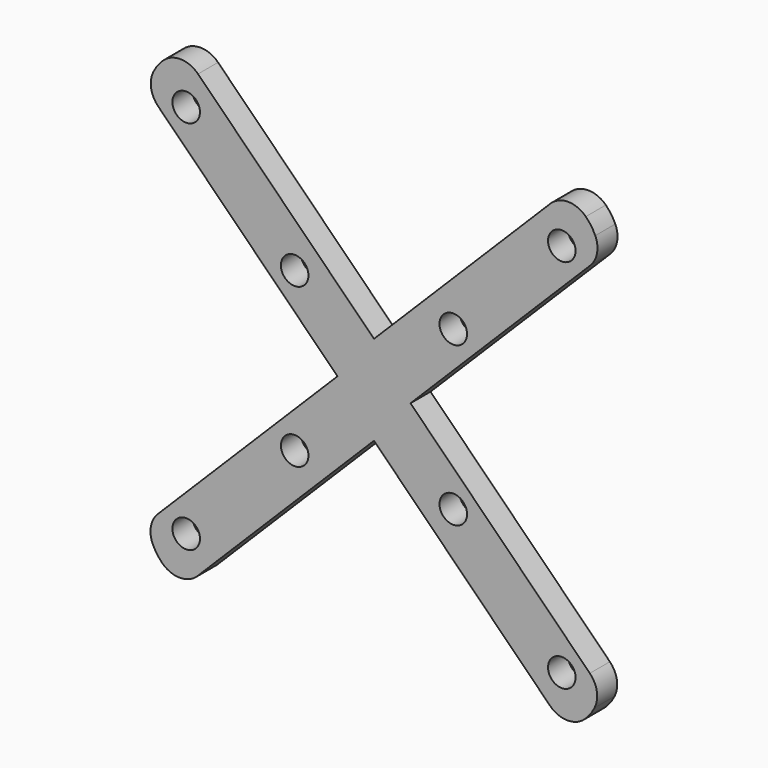
from build123d import *

# Parameters (mm, degrees)
F0_W        = 54
F0_H        = 56
F1_DEPTH    = 3
F3_D        = 3.3
F3_DEPTH    = 4.55
F3_TIP      = 0.9914200214
F5_DEPTH    = 3.001
F7_D        = 3.3
F7_DEPTH    = 4.55
F7_TIP      = 0.9914200214
F8_T1_DEPTH = 29.9160411803
F8_T3_DEPTH = 30.4926194226
F8_T5_DEPTH = 30.4926194226
F8_T7_DEPTH = 29.9160411803
F9_R        = 3


# Not quite as in the source:
# - a fillet or chamfer that OpenCascade refuses, or shapes differently, is made with other operations: its cross-section is extruded or revolved along the edge and cut away or added


with BuildPart() as f1:
    # F0 (on Front) → F1 (new body)
    with BuildSketch(Plane.XZ):
        Rectangle(F0_W, F0_H)
    extrude(amount=F1_DEPTH)

    # F3
    with Locations(Plane.XZ.offset(3)):
        with Locations((-22.5, 22.5), (22.5, 22.5), (22.5, -22.5), (-22.5, -22.5)):
            Hole(F3_D / 2, depth=F3_DEPTH)
            with Locations((0, 0, -(F3_DEPTH + F3_TIP / 2))):  # 118° drill point
                Cone(0, F3_D / 2, F3_TIP, mode=Mode.SUBTRACT)

    # F4 (on face) → F5 (cut, through all)
    with BuildSketch(Plane.XZ.offset(3)):
        Polygon((-4.372583002, 0), (-27, 22.627416998), (-27, -22.627416998), align=None)
        Polygon((22.627416998, 28), (-22.627416998, 28), (0, 5.372583002), align=None)
        Polygon((27, -22.627416998), (27, 22.627416998), (4.372583002, 0), align=None)
        Polygon((0, -5.372583002), (-22.627416998, -28), (22.627416998, -28), align=None)
    extrude(amount=-F5_DEPTH, mode=Mode.SUBTRACT)

    # F7
    with Locations(Plane.XZ.offset(3)):
        with Locations((-9.5, 9.5), (9.5, 9.5), (9.5, -9.5), (-9.5, -9.5)):
            Hole(F7_D / 2, depth=F7_DEPTH)
            with Locations((0, 0, -(F7_DEPTH + F7_TIP / 2))):  # 118° drill point
                Cone(0, F7_D / 2, F7_TIP, mode=Mode.SUBTRACT)

    # F8: fillet of radius 5.5 on 4 edges, made by hand

    # F8_s2 → F8_t1 (cut)
    with BuildSketch(Plane.XZ.offset(-13.4580205902)):
        with BuildLine():
            ThreePointArc((-22.627416998, -28), (-25.7691213082, -26.0844427348), (-27, -22.6167917639))
            Line((-27, -22.6167917639), (-27, -28))
            Line((-27, -28), (-22.627416998, -28))
        make_face()
    extrude(amount=F8_T1_DEPTH, mode=Mode.SUBTRACT)

    # F8_s4 → F8_t3 (cut)
    with BuildSketch(Plane.XZ.offset(-13.7463097113)):
        with BuildLine():
            ThreePointArc((-27, 22.627416998), (-25.3452507259, 26.4338780795), (-21.5014761155, 28))
            Line((-21.5014761155, 28), (-27, 28))
            Line((-27, 28), (-27, 22.627416998))
        make_face()
    extrude(amount=F8_T3_DEPTH, mode=Mode.SUBTRACT)

    # F8_s6 → F8_t5 (cut)
    with BuildSketch(Plane.XZ.offset(-13.7463097113)):
        with BuildLine():
            ThreePointArc((27, -22.627416998), (25.3452507259, -26.4338780795), (21.5014761155, -28))
            Line((21.5014761155, -28), (27, -28))
            Line((27, -28), (27, -22.627416998))
        make_face()
    extrude(amount=F8_T5_DEPTH, mode=Mode.SUBTRACT)

    # F8_s8 → F8_t7 (cut)
    with BuildSketch(Plane.XZ.offset(-13.4580205902)):
        with BuildLine():
            ThreePointArc((22.627416998, 28), (25.7691213082, 26.0844427348), (27, 22.6167917639))
            Line((27, 22.6167917639), (27, 28))
            Line((27, 28), (22.627416998, 28))
        make_face()
    extrude(amount=F8_T7_DEPTH, mode=Mode.SUBTRACT)

    # F9
    f9_edges = [f1.edges().sort_by_distance(p)[0] for p in [
        (-27, -1.5, 22.627417),
        (-26.99999, -1.5, -22.627407),
        (27, -1.5, -22.627417),
        (26.99999, -1.5, 22.627407),
        (-22.627417, -1.5, -28),
        (22.530329, -1.5, -27.902912),
        (-22.530329, -1.5, 27.902912),
        (22.627417, -1.5, 28),
    ]]
    fillet(f9_edges, radius=F9_R)


solid = f1.part
